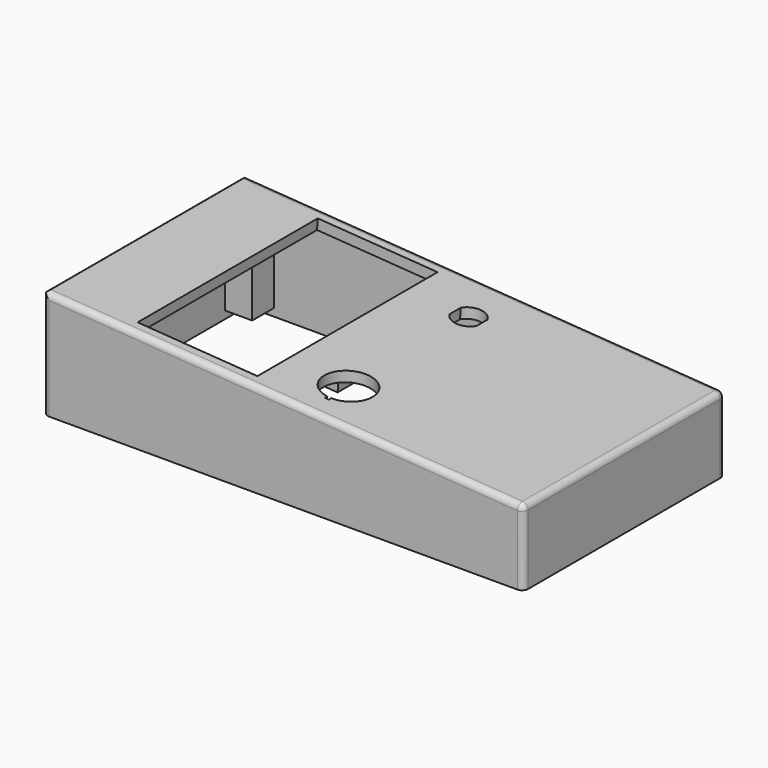
from build123d import *

# Parameters (mm, degrees)
F1_DEPTH      = 42
F2_T          = -3.5
F3_W          = 40
F3_H          = 75
F4_DEPTH      = 4
F6_DEPTH      = 5
F8_W          = 9
F8_H          = 9
F9_DEPTH      = 20.5
F10_DEPTH     = 32
F12_R         = 6
F13_DEPTH     = 25
F15_W         = 8.3580343053
F15_H         = 30.4632759653
F15_W_2       = 12.1421813965
F15_H_2       = 30.5070821196
F16_DEPTH     = 6
F17_T1_DEPTH  = 169.3882617949
F17_T3_DEPTH  = 92.6602540378
F17_T5_DEPTH  = 46.118363099
F17_T7_DEPTH  = 35
F18_D         = 2.5
F18_DEPTH     = 18
F18_TIP       = 0.7510757738
F19_T1_DEPTH  = 80
F19_T6_DEPTH  = 2
F19_T12_DEPTH = 2
F20_D         = 2.5
F20_DEPTH     = 18
F20_TIP       = 0.7510757738


# Not quite as in the source:
# - a fillet or chamfer that OpenCascade refuses, or shapes differently, is made with other operations: its cross-section is extruded or revolved along the edge and cut away or added
# - a feature names something its author has since deleted; it is built from what else it names


with BuildPart() as f1:
    # F0 (on Front) → F1 (new body, symmetric)
    with BuildSketch(Plane.XZ):
        Polygon((-66.6393345791, 36.118363099), (-66.6393345791, 0), (93.3606654209, 0), (93.3606654209, 25), (-65.6393345791, 36.118363099), align=None)
    extrude(amount=F1_DEPTH, both=True)

    # F2
    f2_openings = [f1.faces().sort_by_distance(p)[0] for p in [
        (13.360665, 0, 0),
    ]]
    offset(amount=F2_T, openings=f2_openings)

    # F3 (on face) → F4 (cut)
    with BuildSketch(Plane(origin=(2.1939535511, 0, 31.3749975164), x_dir=(0.9975640503, 0, -0.0697564737), z_dir=(0.0697564737, 0, 0.9975640503))):
        with Locations((-20.9989301063, 0)):
            Rectangle(F3_W, F3_H)
    extrude(amount=-F4_DEPTH, mode=Mode.SUBTRACT)

    # F3 (on face) → F6 (cut)
    with BuildSketch(Plane(origin=(2.1939535511, 0, 31.3749975164), x_dir=(0.9975640503, 0, -0.0697564737), z_dir=(0.0697564737, 0, 0.9975640503))):
        with BuildLine():
            Line((14.9393316886, 27.279802623), (14.9393316886, 22.720197377))
            ThreePointArc((14.9393316886, 22.720197377), (19.3893316886, 20), (23.8393316886, 22.720197377))
            Line((23.8393316886, 22.720197377), (23.8393316886, 27.279802623))
            ThreePointArc((23.8393316886, 27.279802623), (19.3893316886, 30), (14.9393316886, 27.279802623))
        make_face()
        with BuildLine():
            Line((20.0393316886, -34.0238362551), (20.0393316886, -33.0238362551))
            ThreePointArc((20.0393316886, -33.0238362551), (19.3893316886, -16.9498789917), (18.7393316886, -33.0238362551))
            Line((18.7393316886, -33.0238362551), (18.7393316886, -34.0238362551))
            Line((18.7393316886, -34.0238362551), (20.0393316886, -34.0238362551))
        make_face()
    extrude(amount=-F6_DEPTH, mode=Mode.SUBTRACT)

    # F8 (on offset) → F9 (join)
    with BuildSketch(Plane(origin=(0, 0, 2.5), x_dir=(1, 0, 0), z_dir=(0, 0, -1))):
        with Locations((81.6606654209, 34)):
            Rectangle(F8_W, F8_H)
        with Locations((81.6606654209, -34)):
            Rectangle(F8_W, F8_H)
    extrude(amount=-F9_DEPTH)

    # F8 (on offset) → F10 (join)
    with BuildSketch(Plane(origin=(0, 0, 2.5), x_dir=(1, 0, 0), z_dir=(0, 0, -1))):
        with Locations((-58.6393345791, -34)):
            Rectangle(F8_W, F8_H)
        with Locations((-58.6393345791, 34)):
            Rectangle(F8_W, F8_H)
    extrude(amount=-F10_DEPTH)

    # F12 (on offset) → F13 (cut)
    with BuildSketch(Plane(origin=(-66.6393345791, 0, 0), x_dir=(0, -1, 0), z_dir=(-1, 0, 0))):
        with Locations((-22, 23)):
            Circle(F12_R)
        with Locations((22, 23)):
            Circle(F12_R)
    extrude(amount=-F13_DEPTH, mode=Mode.SUBTRACT)

    # F15 (on offset) → F16 (join)
    with BuildSketch(Plane(origin=(1.949805893, 0, 27.8835233405), x_dir=(0.9975640503, 0, -0.0697564737), z_dir=(-0.0697564737, 0, -0.9975640503))):
        with Locations((5.292899441, 1.1196539272)):
            Rectangle(F15_W, F15_H)
        with Locations((44.2803874612, 1.1346279643)):
            Rectangle(F15_W_2, F15_H_2)
    extrude(amount=F16_DEPTH)

    # F17: fillet of radius 2 on 7 edges, made by hand

    # F17_s2 → F17_t1 (cut)
    with BuildSketch(Plane(origin=(96.1545321211, 0, -6.7237798852), x_dir=(0, 1, 0), z_dir=(-0.9975640503, 0, 0.0697564737))):
        with BuildLine():
            ThreePointArc((40, -31.4516120627), (41.4142135624, -30.865825625), (42, -29.4516120627))
            Line((42, -29.4516120627), (42, -31.4516120627))
            Line((42, -31.4516120627), (40, -31.4516120627))
        make_face()
        with BuildLine():
            ThreePointArc((-40, -31.4516120627), (-41.4142135624, -30.865825625), (-42, -29.4516120627))
            Line((-42, -29.4516120627), (-42, -31.4516120627))
            Line((-42, -31.4516120627), (-40, -31.4516120627))
        make_face()
    extrude(amount=F17_T1_DEPTH, mode=Mode.SUBTRACT)

    # F17_s4 → F17_t3 (cut)
    with BuildSketch(Plane.XZ.offset(-46.3301270189)):
        with BuildLine():
            ThreePointArc((-65.6393345791, 36.118363099), (-66.3713853867, 35.3863122914), (-66.6393345791, 34.3863122914))
            Line((-66.6393345791, 34.3863122914), (-66.6393345791, 36.118363099))
            Line((-66.6393345791, 36.118363099), (-65.6393345791, 36.118363099))
        make_face()
    extrude(amount=F17_T3_DEPTH, mode=Mode.SUBTRACT)

    # F17_s6 → F17_t5 (cut)
    with BuildSketch(Plane.XY.offset(-5)):
        with BuildLine():
            ThreePointArc((-64.6393345791, 42), (-66.0535481415, 41.4142135624), (-66.6393345791, 40))
            Line((-66.6393345791, 40), (-66.6393345791, 42))
            Line((-66.6393345791, 42), (-64.6393345791, 42))
        make_face()
        with BuildLine():
            ThreePointArc((-64.6393345791, -42), (-66.0535481415, -41.4142135624), (-66.6393345791, -40))
            Line((-66.6393345791, -40), (-66.6393345791, -42))
            Line((-66.6393345791, -42), (-64.6393345791, -42))
        make_face()
    extrude(amount=F17_T5_DEPTH, mode=Mode.SUBTRACT)

    # F17_s8 → F17_t7 (cut)
    with BuildSketch(Plane.XY.offset(-5)):
        with BuildLine():
            ThreePointArc((91.3606654209, 42), (92.7748789833, 41.4142135624), (93.3606654209, 40))
            Line((93.3606654209, 40), (93.3606654209, 42))
            Line((93.3606654209, 42), (91.3606654209, 42))
        make_face()
        with BuildLine():
            ThreePointArc((93.3606654209, -40), (92.7748789833, -41.4142135624), (91.3606654209, -42))
            Line((91.3606654209, -42), (93.3606654209, -42))
            Line((93.3606654209, -42), (93.3606654209, -40))
        make_face()
    extrude(amount=F17_T7_DEPTH, mode=Mode.SUBTRACT)

    # F18
    with Locations(Plane(origin=(0, 0, 2.5), x_dir=(1, 0, 0), z_dir=(0, 0, -1))):
        with Locations((-58.6393345791, 34), (-58.6393345791, -34)):
            Hole(F18_D / 2, depth=F18_DEPTH)
            with Locations((0, 0, -(F18_DEPTH + F18_TIP / 2))):  # 118° drill point
                Cone(0, F18_D / 2, F18_TIP, mode=Mode.SUBTRACT)

    # F19: fillet of radius 2 on 1 edges, made by hand

    # F19_s2 → F19_t1 (cut)
    with BuildSketch(Plane.XZ.offset(-40)):
        with BuildLine():
            ThreePointArc((91.5001783684, 25.1300979282), (92.8233728241, 24.4989665478), (93.3606654209, 23.1349698277))
            Line((93.3606654209, 23.1349698277), (93.3606654209, 25))
            Line((93.3606654209, 25), (91.5001783684, 25.1300979282))
        make_face()
    extrude(amount=F19_T1_DEPTH, mode=Mode.SUBTRACT)


with BuildPart() as f19_tool4:
    # F19_s5 → F19_t6 (new body)
    with BuildSketch(Plane.XZ.offset(40)):
        Polygon((91.3606654209, 23.1349698277), (91.5001783684, 25.1300979282), (93.3606654209, 25), (93.3606654209, 23.1349698277), align=None)
    extrude(amount=F19_T6_DEPTH)

    # F19_s7 → F19_t8 (revolve, cut)
    with BuildSketch(Plane(origin=(91.3606654209, -40, 23.1349698277), x_dir=(-0.7313537016, 0, -0.6819983601), z_dir=(-0.6819983601, 0, 0.7313537016))):
        with BuildLine():
            ThreePointArc((0, -2), (2, 0), (0, 2))
            Line((0, 2), (0, -2))
        make_face()
    revolve(axis=Axis((91.3606654209, -40, 23.1349698277), (0, -1, 0)), mode=Mode.SUBTRACT)


with BuildPart() as f1_1:
    add(f1.part)

    # F19_t3: cut F19_tool4
    add(f19_tool4.part, mode=Mode.SUBTRACT)


with BuildPart() as f19_tool10:
    # F19_s11 → F19_t12 (new body)
    with BuildSketch(Plane.XZ.offset(-40)):
        Polygon((91.3606654209, 23.1349698277), (91.5001783684, 25.1300979282), (93.3606654209, 25), (93.3606654209, 23.1349698277), align=None)
    extrude(amount=-F19_T12_DEPTH)

    # F19_s13 → F19_t14 (revolve, cut)
    with BuildSketch(Plane(origin=(91.3606654209, 40, 23.1349698277), x_dir=(-0.7313537016, 0, -0.6819983601), z_dir=(0.6819983601, 0, -0.7313537016))):
        with BuildLine():
            ThreePointArc((0, -2), (2, 0), (0, 2))
            Line((0, 2), (0, -2))
        make_face()
    revolve(axis=Axis((91.3606654209, 40, 23.1349698277), (0, 1, 0)), mode=Mode.SUBTRACT)


with BuildPart() as f1_2:
    add(f1_1.part)

    # F19_t9: cut F19_tool10
    add(f19_tool10.part, mode=Mode.SUBTRACT)

    # F20
    with Locations(Plane(origin=(0, 0, 2.5), x_dir=(1, 0, 0), z_dir=(0, 0, -1))):
        with Locations((81.6606654209, 34), (81.6606654209, -34)):
            Hole(F20_D / 2, depth=F20_DEPTH)
            with Locations((0, 0, -(F20_DEPTH + F20_TIP / 2))):  # 118° drill point
                Cone(0, F20_D / 2, F20_TIP, mode=Mode.SUBTRACT)


solid = f1_2.part
